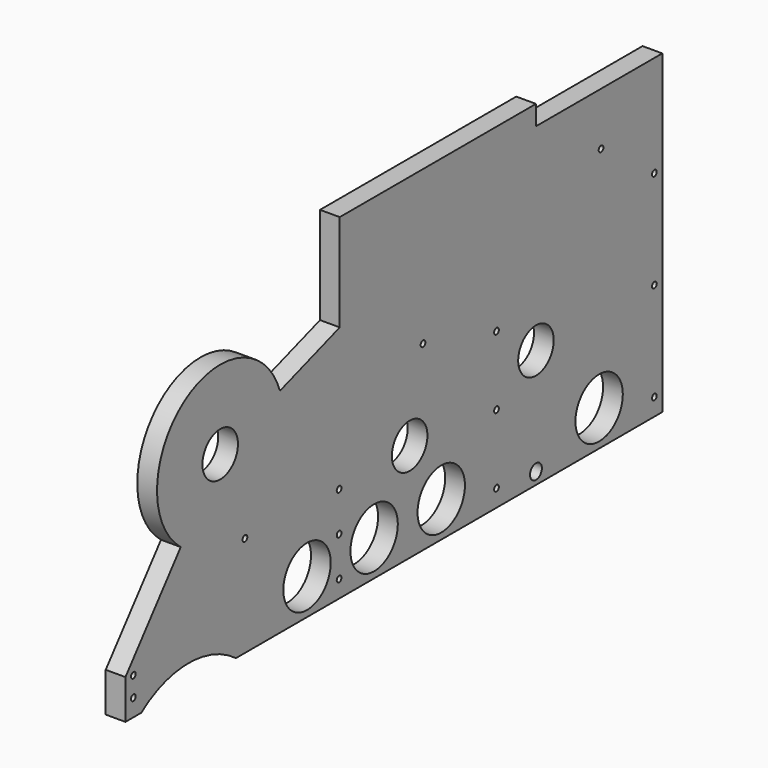
from build123d import *

# Parameters (mm, degrees)
F0_R     = 1.905
F0_R_2   = 14.2875
F0_R_3   = 4.7625
F1_DEPTH = 12.7
F2_R     = 19.05
F3_DEPTH = 12.7
F5_DEPTH = 12.7
F6_R     = 1.905
F7_DEPTH = 12.7


with BuildPart() as f1:
    # F0 (on Right) → F1 (new body)
    with BuildSketch(Plane.YZ):
        with BuildLine():
            Line((0, 355.6), (0, 0))
            Line((0, 0), (12.7, 0))
            ThreePointArc((12.7, 0), (50.8, 12.7), (88.9, 0))
            Line((88.9, 0), (431.8, 0))
            Line((431.8, 0), (431.8, 355.6))
            Line((431.8, 355.6), (0, 355.6))
        make_face()
        with Locations((96.1134966165, 64.8649486739)):
            Circle(F0_R, mode=Mode.SUBTRACT)
        with Locations((228.6, 63.5)):
            Circle(F0_R_2, mode=Mode.SUBTRACT)
        with Locations((239.3226520243, 116.9888185167)):
            Circle(F0_R, mode=Mode.SUBTRACT)
        with Locations((330.2, 7.62)):
            Circle(F0_R_3, mode=Mode.SUBTRACT)
        with Locations((330.2, 76.2)):
            Circle(F0_R_2, mode=Mode.SUBTRACT)
        with Locations((76.2, 120.65)):
            Circle(F0_R_2, mode=Mode.SUBTRACT)
        with Locations((382.531807432, 169.1126883595)):
            Circle(F0_R, mode=Mode.SUBTRACT)
    extrude(amount=F1_DEPTH)

    # F2 (on face) → F3 (cut, through all)
    with BuildSketch(Plane.YZ.offset(12.7)):
        with Locations((146.05, 23.05)):
            Circle(F2_R)
        with Locations((254, 23.05)):
            Circle(F2_R)
        with Locations((381, 23.0378)):
            Circle(F2_R)
        with Locations((200.025, 23.05)):
            Circle(F2_R)
    extrude(amount=-F3_DEPTH, mode=Mode.SUBTRACT)

    # F4 (on face) → F5 (cut, through all)
    with BuildSketch(Plane.YZ.offset(12.7)):
        Polygon((431.8, 355.6), (0, 355.6), (0, 215.9), (172.3654351189, 215.9), (330.2, 215.9), (355.6, 215.9), (431.8, 215.9), align=None)
        with BuildLine():
            Line((172.3654351189, 215.9), (0, 215.9))
            Line((0, 215.9), (0, 25.4))
            Line((0, 25.4), (44.4654915842, 80.9818644803))
            ThreePointArc((44.4654915842, 80.9818644803), (47.0024645882, 162.2209505049), (124.2827175595, 137.0418355316))
            Line((124.2827175595, 137.0418355316), (172.3654351189, 153.4336710633))
            Line((172.3654351189, 153.4336710633), (172.3654351189, 215.9))
        make_face()
        Polygon((431.8, 203.2), (431.8, 215.9), (355.6, 215.9), (330.2, 207.2409090909), (330.2, 203.2), align=None)
        Polygon((330.2, 207.2409090909), (355.6, 215.9), (330.2, 215.9), align=None)
    extrude(amount=-F5_DEPTH, mode=Mode.SUBTRACT)

    # F6 (on face) → F7 (cut, through all)
    with BuildSketch(Plane.YZ.offset(12.7)):
        with Locations((425.45, 11.1125)):
            Circle(F6_R)
        with Locations((425.45, 74.5109)):
            Circle(F6_R)
        with Locations((425.45, 137.9093)):
            Circle(F6_R)
        with Locations((298.45, 11.1125)):
            Circle(F6_R)
        with Locations((298.45, 100.0125)):
            Circle(F6_R)
        with Locations((298.45, 55.5625)):
            Circle(F6_R)
        with Locations((171.8554794788, 11.1125)):
            Circle(F6_R)
        with Locations((171.8554794788, 36.5125)):
            Circle(F6_R)
        with Locations((171.8554794788, 61.9125)):
            Circle(F6_R)
        with Locations((6.35, 11.1125)):
            Circle(F6_R)
        with Locations((6.35, 23.8125)):
            Circle(F6_R)
    extrude(amount=-F7_DEPTH, mode=Mode.SUBTRACT)


solid = f1.part
